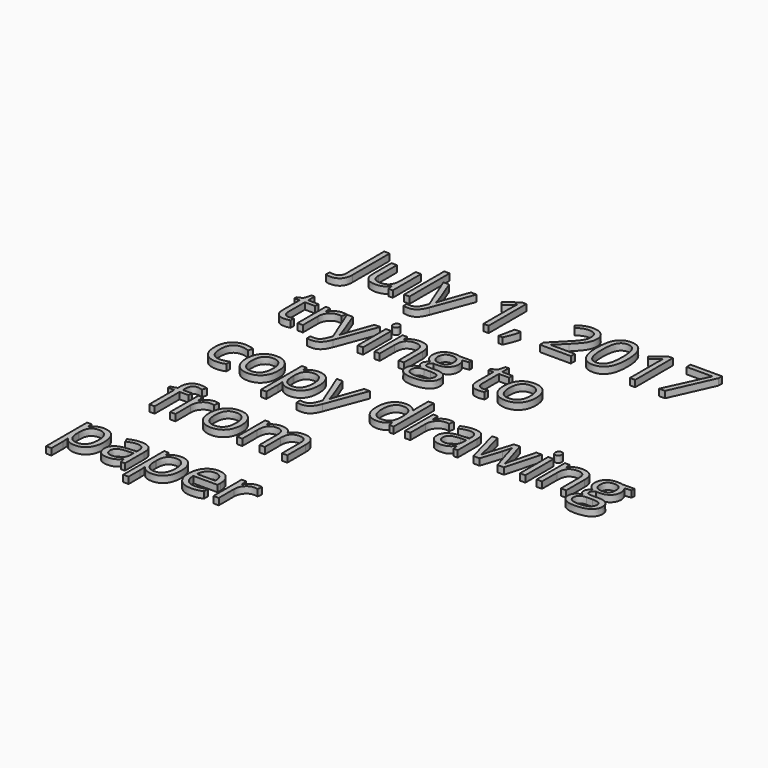
from build123d import *

# Parameters (mm, degrees)
F0_TEXT_SIZE = 255.7638888889
F1_DEPTH     = 25.4


# Not quite as in the source:
# - Text() gives the source's letters only with a copy of the font that has no kerning and outlines rounded to 1/6400 em; it was checked with that copy


with BuildPart() as f1:
    # F0 (on Top) → F1 (new body)
    with BuildSketch(Plane.XY):
        with Locations((76.3823567301, -152.1553844531)):
            Text('July 1, 2017', F0_TEXT_SIZE, font='Open Sans', text_align=(TextAlign.LEFT, TextAlign.BOTTOM))
        with Locations((76.3823567301, -499.994273342)):
            Text('trying to', F0_TEXT_SIZE, font='Open Sans', text_align=(TextAlign.LEFT, TextAlign.BOTTOM))
        with Locations((76.3823567301, -847.8331622309)):
            Text('copy drawing', F0_TEXT_SIZE, font='Open Sans', text_align=(TextAlign.LEFT, TextAlign.BOTTOM))
        with Locations((142.8410047336, -1195.6720511198)):
            Text('from', F0_TEXT_SIZE, font='Open Sans', text_align=(TextAlign.LEFT, TextAlign.BOTTOM))
        with Locations((76.3823567301, -1543.5109400087)):
            Text('paper', F0_TEXT_SIZE, font='Open Sans', text_align=(TextAlign.LEFT, TextAlign.BOTTOM))
    extrude(amount=F1_DEPTH)


solid = f1.part
